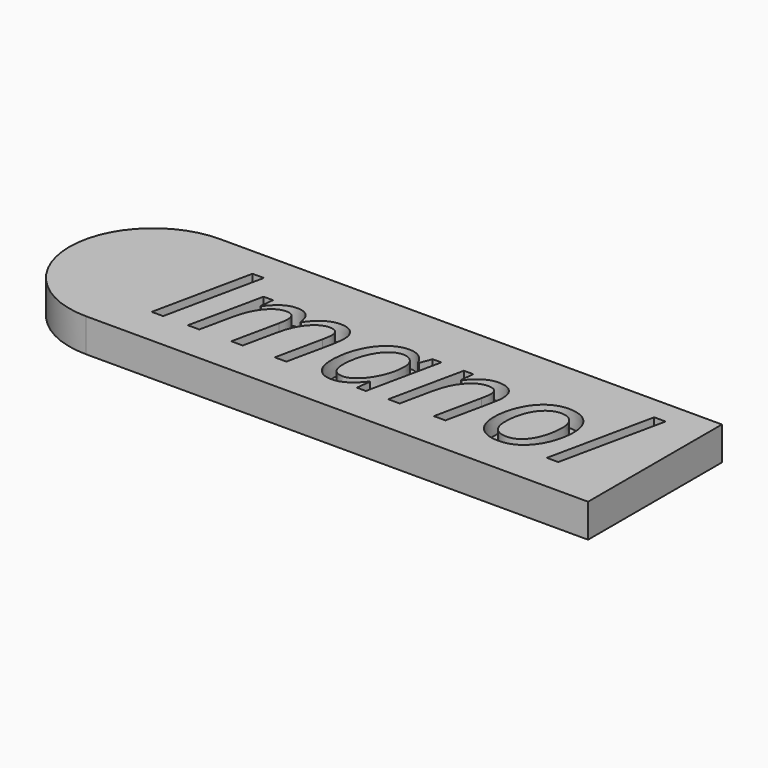
from build123d import *

# Parameters (mm, degrees)
F1_DEPTH     = 4
F2_TEXT_SIZE = 16.6666666667
F3_DEPTH     = 2


# Not quite as in the source:
# - Text() gives the source's letters only with a copy of the font that has no kerning and outlines rounded to 1/6400 em; it was checked with that copy


with BuildPart() as f1:
    # F0 (on Top) → F1 (new body)
    with BuildSketch(Plane.XY):
        with BuildLine():
            Line((30, -10), (30, 10))
            Line((30, 10), (-30, 10))
            ThreePointArc((-30, 10), (-40, 0), (-30, -10))
            Line((-30, -10), (30, -10))
        make_face()
    extrude(amount=F1_DEPTH)

    # F2 (on face) → F3 (cut)
    with BuildSketch(Plane.XY.offset(4)):
        with Locations((-26.484422803, -5.4792037078)):
            Text('Imanol', F2_TEXT_SIZE, font='Open Sans', font_style=FontStyle.ITALIC, text_align=(TextAlign.LEFT, TextAlign.BOTTOM))
    extrude(amount=-F3_DEPTH, mode=Mode.SUBTRACT)


solid = f1.part
